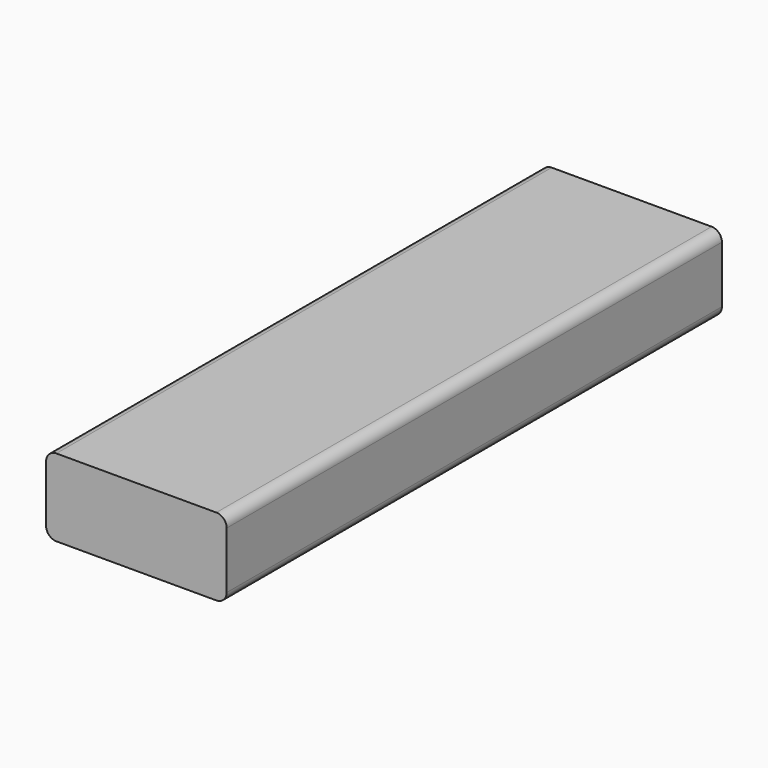
from build123d import *

# Parameters (mm, degrees)
F0_W     = 88.9
F0_H     = 304.8
F1_DEPTH = 38.1
F2_R     = 5.08
F3_R     = 5.08


# Not quite as in the source:
# - a feature names something its author has since deleted; it is built from what else it names


with BuildPart() as f1:
    # F0 (on Top) → F1 (new body)
    with BuildSketch(Plane.XY):
        with Locations((44.45, -152.4)):
            Rectangle(F0_W, F0_H)
    extrude(amount=F1_DEPTH)

    # F2
    f2_edges = [f1.edges().sort_by_distance(p)[0] for p in [
        (0, -152.4, 38.1),
        (0, -152.4, 0),
    ]]
    fillet(f2_edges, radius=F2_R)

    # F3
    f3_edges = [f1.edges().sort_by_distance(p)[0] for p in [
        (88.9, -152.4, 38.1),
        (88.9, -152.4, 0),
    ]]
    fillet(f3_edges, radius=F3_R)


solid = f1.part
